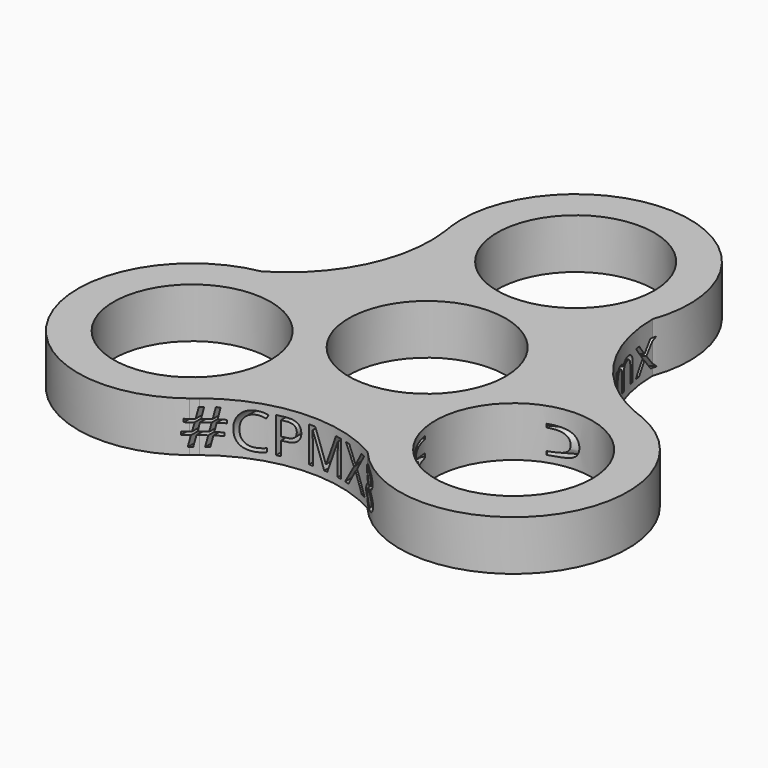
from build123d import *

# Parameters (mm, degrees)
F0_R         = 11
F1_DEPTH     = 7
F3_TEXT_SIZE = 6.9444444444
F4_DEPTH     = 15
F7_TEXT_SIZE = 6.9444444444
F8_DEPTH     = 25


# Not quite as in the source:
# - Text() gives the source's letters only with a copy of the font that has no kerning and outlines rounded to 1/6400 em; it was checked with that copy


with BuildPart() as f1:
    # F0 (on Top) → F1 (new body)
    with BuildSketch(Plane.XY):
        with BuildLine():
            ThreePointArc((27.5673724722, 2.1819072767), (18.5138998492, 9.4958807108), (15.0655062663, 20.61200214))
            ThreePointArc((15.0655062663, 20.61200214), (1.6861353643, 41.9109065591), (-15.8601693175, 23.8893059864))
            ThreePointArc((-15.8601693175, 23.8893059864), (-15.7589632332, 23.3375093516), (-15.6732733664, 22.7830912382))
            ThreePointArc((-15.6732733664, 22.7830912382), (-17.4806238514, 11.2855672371), (-25.3832706093, 2.7411100775))
            ThreePointArc((-25.3832706093, 2.7411100775), (-37.138977458, -19.4952172199), (-12.7586612042, -25.6799625305))
            ThreePointArc((-12.7586612042, -25.6799625305), (-12.3313943429, -25.3164171731), (-11.8940991058, -24.9649985149))
            ThreePointArc((-11.8940991058, -24.9649985149), (-1.0332759977, -20.7814479479), (10.317764343, -23.3531122175))
            ThreePointArc((10.317764343, -23.3531122175), (35.4528420937, -22.4156893392), (28.6188305218, 1.7906565441))
            ThreePointArc((28.6188305218, 1.7906565441), (28.0903575761, 1.9789078215), (27.5673724722, 2.1819072767))
        make_face()
        with Locations((-22.5166604984, -13)):
            Circle(F0_R, mode=Mode.SUBTRACT)
        with Locations((22.5166604984, -13)):
            Circle(F0_R, mode=Mode.SUBTRACT)
        Circle(F0_R, mode=Mode.SUBTRACT)
        with Locations((0, 26)):
            Circle(F0_R, mode=Mode.SUBTRACT)
    extrude(amount=F1_DEPTH)

    # F3 (on offset) → F4 (cut)
    with BuildSketch(Plane.XZ.offset(30)):
        with Locations((-13.6935763889, 1)):
            Text('#CPMX8', F3_TEXT_SIZE, font='Open Sans', text_align=(TextAlign.LEFT, TextAlign.BOTTOM))
    extrude(amount=-F4_DEPTH, mode=Mode.SUBTRACT)

    # F7 (on face) → F8 (cut)
    with BuildSketch(Plane(origin=(34.6410161514, 20, 0), x_dir=(-0.5, 0.8660254038, 0), z_dir=(0.8660254038, 0.5, 0))):
        with Locations((-13.5903136999, 1)):
            Text('d3d.mx', F7_TEXT_SIZE, font='Open Sans', text_align=(TextAlign.LEFT, TextAlign.BOTTOM))
    extrude(amount=-F8_DEPTH, mode=Mode.SUBTRACT)


solid = f1.part
